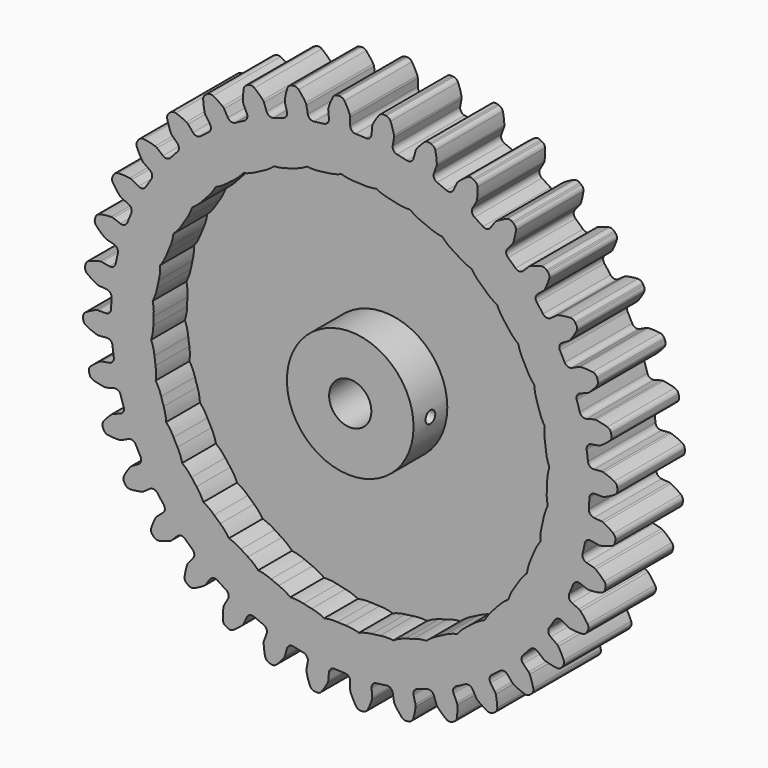
from build123d import *

# Parameters (mm, degrees)
F1_DEPTH = 12.7
F2_R     = 3.175
F3_DEPTH = 12.701
F4_T     = -6.35
F6_R     = 0.9144
F7_DEPTH = 9.525


# Not quite as in the source:
# - a shell that OpenCascade refuses in one call is made with other operations: the cavity is built on its own and cut out


with BuildPart() as f1:
    # F0 (on Front) → F1 (new body)
    with BuildSketch(Plane.XZ):
        with BuildLine():
            ThreePointArc((0, 37.9424051819), (-0.0153371145, 38.1007918887), (-0.0607785558, 38.2532932047))
            ThreePointArc((-0.0607785558, 38.2532932047), (-0.4269499275, 39.0474115053), (-0.8644079312, 39.8046009426))
            ThreePointArc((-0.8644079312, 39.8046009426), (-1.1764211516, 40.0905083584), (-1.58910835, 40.18423443))
            Line((-1.58910835, 40.18423443), (-1.7542226688, 40.1783047252))
            Line((-1.7542226688, 40.1783047252), (-1.9192254855, 40.1698212046))
            ThreePointArc((-1.9192254855, 40.1698212046), (-2.3221735191, 40.0404837297), (-2.6080809619, 39.7284705339))
            ThreePointArc((-2.6080809619, 39.7284705339), (-2.977880898, 38.9360354539), (-3.2734469068, 38.1130250753))
            ThreePointArc((-3.2734469068, 38.1130250753), (-3.3054240642, 37.9571435902), (-3.3068985053, 37.798022875))
            Line((-3.3068985053, 37.798022875), (-3.2072574352, 36.6591202325))
            ThreePointArc((-3.2072574352, 36.6591202325), (-3.3913357559, 36.0636768654), (-3.9392441989, 35.7666348321))
            Line((-3.9392441989, 35.7666348321), (-5.452068566, 35.5674677257))
            ThreePointArc((-5.452068566, 35.5674677257), (-6.058187617, 35.7125791572), (-6.3901057047, 36.2400903084))
            Line((-6.3901057047, 36.2400903084), (-6.5886295161, 37.365974791))
            ThreePointArc((-6.5886295161, 37.365974791), (-6.6312371884, 37.5192919859), (-6.7024698477, 37.6615856408))
            ThreePointArc((-6.7024698477, 37.6615856408), (-7.2009754492, 38.3800545087), (-7.7632720488, 39.0497767518))
            ThreePointArc((-7.7632720488, 39.0497767518), (-8.1201923891, 39.2771600644), (-8.5428853032, 39.2977998464))
            Line((-8.5428853032, 39.2977998464), (-8.704461482, 39.2632884266))
            Line((-8.704461482, 39.2632884266), (-8.8654843873, 39.2262813513))
            ThreePointArc((-8.8654843873, 39.2262813513), (-9.239851518, 39.0289376116), (-9.4672348615, 38.6720172909))
            ThreePointArc((-9.4672348615, 38.6720172909), (-9.6938117981, 37.8274059953), (-9.8419732426, 36.9655744948))
            ThreePointArc((-9.8419732426, 36.9655744948), (-9.8463960593, 36.8065084247), (-9.8202170781, 36.6495490767))
            Line((-9.8202170781, 36.6495490767), (-9.5243214113, 35.5452514147))
            ThreePointArc((-9.5243214113, 35.5452514147), (-9.6022055131, 34.9268893053), (-10.090209188, 34.5392167052))
            Line((-10.090209188, 34.5392167052), (-11.5454653485, 34.0803762003))
            ThreePointArc((-11.5454653485, 34.0803762003), (-12.1675744249, 34.1180315944), (-12.5860512811, 34.5798916949))
            Line((-12.5860512811, 34.5798916949), (-12.9770668584, 35.6541981643))
            ThreePointArc((-12.9770668584, 35.6541981643), (-13.0456504759, 35.7977873818), (-13.1405099849, 35.9255498549))
            ThreePointArc((-13.1405099849, 35.9255498549), (-13.7562029759, 36.546538977), (-14.4262530737, 37.1084448546))
            ThreePointArc((-14.4262530737, 37.1084448546), (-14.8172356899, 37.2703951371), (-15.2370910093, 37.2173215002))
            Line((-15.2370910093, 37.2173215002), (-15.3902196378, 37.1552769774))
            Line((-15.3902196378, 37.1552769774), (-15.5423700321, 37.0908707886))
            ThreePointArc((-15.5423700321, 37.0908707886), (-15.8767813042, 36.8315169737), (-16.0387316204, 36.4405343714))
            ThreePointArc((-16.0387316204, 36.4405343714), (-16.1152011319, 35.5694099471), (-16.1114562016, 34.6949436388))
            ThreePointArc((-16.1114562016, 34.6949436388), (-16.0881902927, 34.5375261256), (-16.0351533242, 34.3874972752))
            Line((-16.0351533242, 34.3874972752), (-15.5519937009, 33.3513581193))
            ThreePointArc((-15.5519937009, 33.3513581193), (-15.5213171147, 32.7288658876), (-15.9345882767, 32.2623419565))
            ThreePointArc((-15.9345882767, 32.2623419565), (-16.6150587927, 31.9172309793), (-17.2880590087, 31.5577696895))
            ThreePointArc((-17.2880590087, 31.5577696895), (-17.9072556409, 31.4868249062), (-18.3995760581, 31.8690005704))
            Line((-18.3995760581, 31.8690005704), (-18.9712025909, 32.8590867682))
            ThreePointArc((-18.9712025909, 32.8590867682), (-19.0636782751, 32.9885851227), (-19.1792823757, 33.0979344158))
            ThreePointArc((-19.1792823757, 33.0979344158), (-19.893455236, 33.6025753519), (-20.6508996989, 34.0395916382))
            ThreePointArc((-20.6508996989, 34.0395916382), (-21.0640647821, 34.1311881132), (-21.4683254155, 34.006013673))
            Line((-21.4683254155, 34.006013673), (-21.6083537576, 33.9183212386))
            Line((-21.6083537576, 33.9183212386), (-21.7470086284, 33.8284728859))
            ThreePointArc((-21.7470086284, 33.8284728859), (-22.0313031244, 33.5149893302), (-22.1228996351, 33.1018242549))
            ThreePointArc((-22.1228996351, 33.1018242549), (-22.0469382341, 32.2306553767), (-21.8914007168, 31.3701244769))
            ThreePointArc((-21.8914007168, 31.3701244769), (-21.841153005, 31.2191385721), (-21.7628695508, 31.08059877))
            Line((-21.7628695508, 31.08059877), (-21.1071265316, 30.1441006842))
            ThreePointArc((-21.1071265316, 30.1441006842), (-20.96882135, 29.5363924414), (-21.294802964, 29.005192273))
            ThreePointArc((-21.294802964, 29.005192273), (-21.9050077115, 28.5471618419), (-22.5053637442, 28.0762963158))
            ThreePointArc((-22.5053637442, 28.0762963158), (-23.1028339558, 27.8989069763), (-23.6540390273, 28.1897859902))
            Line((-23.6540390273, 28.1897859902), (-24.3889079326, 29.0655686481))
            ThreePointArc((-24.3889079326, 29.0655686481), (-24.5024658566, 29.1770413976), (-24.6353019766, 29.2646549879))
            ThreePointArc((-24.6353019766, 29.2646549879), (-25.4262549254, 29.6376144785), (-26.2480791867, 29.9364626548))
            ThreePointArc((-26.2480791867, 29.9364626548), (-26.6708729248, 29.9549222097), (-27.0472556174, 29.7614503283))
            Line((-27.0472556174, 29.7614503283), (-27.169928983, 29.6507744726))
            Line((-27.169928983, 29.6507744726), (-27.2908753719, 29.5382139526))
            ThreePointArc((-27.2908753719, 29.5382139526), (-27.5164149476, 29.1801256953), (-27.5348745391, 28.7573319588))
            ThreePointArc((-27.5348745391, 28.7573319588), (-27.3087902743, 27.9125886522), (-27.0061860988, 27.0921399567))
            ThreePointArc((-27.0061860988, 27.0921399567), (-26.9304833354, 26.9521732907), (-26.8293319986, 26.8293319986))
            Line((-26.8293319986, 26.8293319986), (-26.0209300033, 26.0209300033))
            ThreePointArc((-26.0209300033, 26.0209300033), (-25.7791985593, 25.446470657), (-26.0079858389, 24.8667344996))
            ThreePointArc((-26.0079858389, 24.8667344996), (-26.5293840555, 24.3097016375), (-27.0388543905, 23.7417388857))
            ThreePointArc((-27.0388543905, 23.7417388857), (-27.5964443516, 23.4632948755), (-28.1897859902, 23.6540390273))
            Line((-28.1897859902, 23.6540390273), (-29.0655686481, 24.3889079326))
            ThreePointArc((-29.0655686481, 24.3889079326), (-29.1967584119, 24.478968034), (-29.3427903931, 24.5421838268))
            ThreePointArc((-29.3427903931, 24.5421838268), (-30.1864907252, 24.7721296865), (-31.0477240705, 24.9237294022))
            ThreePointArc((-31.0477240705, 24.9237294022), (-31.4673000898, 24.8684911528), (-31.8043686439, 24.6126003753))
            Line((-31.8043686439, 24.6126003753), (-31.9059596648, 24.4823039282))
            Line((-31.9059596648, 24.4823039282), (-32.0055226772, 24.3504513354))
            ThreePointArc((-32.0055226772, 24.3504513354), (-32.1654544266, 23.958638707), (-32.1102162135, 23.5390626829))
            ThreePointArc((-32.1102162135, 23.5390626829), (-31.7408785409, 22.7464120459), (-31.300402182, 21.9909744733))
            ThreePointArc((-31.300402182, 21.9909744733), (-31.2015445572, 21.8662798623), (-31.08059877, 21.7628695508))
            Line((-31.08059877, 21.7628695508), (-30.1441006842, 21.1071265316))
            ThreePointArc((-30.1441006842, 21.1071265316), (-29.8062878653, 20.5833707383), (-29.9309292248, 19.9727135815))
            ThreePointArc((-29.9309292248, 19.9727135815), (-30.3476784895, 19.3336034502), (-30.7507831285, 18.6858007336))
            ThreePointArc((-30.7507831285, 18.6858007336), (-31.2515507502, 18.3147624328), (-31.8690005704, 18.3995760581))
            Line((-31.8690005704, 18.3995760581), (-32.8590867682, 18.9712025909))
            ThreePointArc((-32.8590867682, 18.9712025909), (-33.0039222371, 19.0371136136), (-33.1587129716, 19.074010829))
            ThreePointArc((-33.1587129716, 19.074010829), (-34.0295252794, 19.1539562693), (-34.9039995693, 19.1537012437))
            ThreePointArc((-34.9039995693, 19.1537012437), (-35.3076092648, 19.0264435763), (-35.595122023, 18.7159090145))
            Line((-35.595122023, 18.7159090145), (-35.6725439074, 18.5699509676))
            Line((-35.6725439074, 18.5699509676), (-35.7476983714, 18.4228125762))
            ThreePointArc((-35.7476983714, 18.4228125762), (-35.8371628493, 18.0091806053), (-35.7099052168, 17.6055708988))
            ThreePointArc((-35.7099052168, 17.6055708988), (-35.2085362747, 16.8890972198), (-34.6435713836, 16.2216243584))
            ThreePointArc((-34.6435713836, 16.2216243584), (-34.5245626363, 16.1159905852), (-34.3874972752, 16.0351533242))
            Line((-34.3874972752, 16.0351533242), (-33.3513581193, 15.5519937009))
            ThreePointArc((-33.3513581193, 15.5519937009), (-32.9277281972, 15.0948555154), (-32.9444364719, 14.471831868))
            ThreePointArc((-32.9444364719, 14.471831868), (-33.2438740692, 13.7700635053), (-33.5283648817, 13.0621039816))
            ThreePointArc((-33.5283648817, 13.0621039816), (-33.9570945933, 12.6097452014), (-34.5798916949, 12.5860512811))
            Line((-34.5798916949, 12.5860512811), (-35.6541981643, 12.9770668584))
            ThreePointArc((-35.6541981643, 12.9770668584), (-35.808278586, 13.0168261293), (-35.9671248356, 13.0262836642))
            ThreePointArc((-35.9671248356, 13.0262836642), (-36.8385899278, 12.9537995833), (-37.6997347036, 12.8016975651))
            ThreePointArc((-37.6997347036, 12.8016975651), (-38.0751145988, 12.6062871396), (-38.3043356314, 12.2505442291))
            Line((-38.3043356314, 12.2505442291), (-38.3552359546, 12.0933594436))
            Line((-38.3552359546, 12.0933594436), (-38.4036983399, 11.9354059794))
            ThreePointArc((-38.4036983399, 11.9354059794), (-38.4199772133, 11.512522664), (-38.2245668202, 11.1371427518))
            ThreePointArc((-38.2245668202, 11.1371427518), (-37.6064004502, 10.518615721), (-36.9341131993, 9.959388396))
            ThreePointArc((-36.9341131993, 9.959388396), (-36.79856935, 9.8760250892), (-36.6495490767, 9.8202170781))
            Line((-36.6495490767, 9.8202170781), (-35.5452514147, 9.5243214113))
            ThreePointArc((-35.5452514147, 9.5243214113), (-35.0486761701, 9.147690746), (-34.9569436875, 8.5312308663))
            ThreePointArc((-34.9569436875, 8.5312308663), (-35.1299713576, 7.7881271488), (-35.2872042343, 7.0415218098))
            ThreePointArc((-35.2872042343, 7.0415218098), (-35.6308693003, 6.5215872428), (-36.2400903084, 6.3901057047))
            Line((-36.2400903084, 6.3901057047), (-37.365974791, 6.5886295161))
            ThreePointArc((-37.365974791, 6.5886295161), (-37.5246185099, 6.6010289699), (-37.6826938117, 6.5827594618))
            ThreePointArc((-37.6826938117, 6.5827594618), (-38.5283326624, 6.3600482518), (-39.3499824758, 6.0607207841))
            ThreePointArc((-39.3499824758, 6.0607207841), (-39.6857268427, 5.8030950472), (-39.8496913846, 5.4129528563))
            Line((-39.8496913846, 5.4129528563), (-39.8725235659, 5.2493173126))
            Line((-39.8725235659, 5.2493173126), (-39.8928213675, 5.0853481115))
            ThreePointArc((-39.8928213675, 5.0853481115), (-39.8354200112, 4.6660625471), (-39.5777943034, 4.3303181579))
            ThreePointArc((-39.5777943034, 4.3303181579), (-38.8616131778, 3.8285314062), (-38.1024306749, 3.3945414568))
            ThreePointArc((-38.1024306749, 3.3945414568), (-37.954470155, 3.3359815684), (-37.798022875, 3.3068985053))
            Line((-37.798022875, 3.3068985053), (-36.6591202325, 3.2072574352))
            ThreePointArc((-36.6591202325, 3.2072574352), (-36.104687853, 2.9225780222), (-35.9073018583, 2.3314127318))
            ThreePointArc((-35.9073018583, 2.3314127318), (-35.9486622428, 1.5695524898), (-35.9738597423, 0.8069865611))
            ThreePointArc((-35.9738597423, 0.8069865611), (-36.2220180737, 0.235274156), (-36.7991521163, 0))
            Line((-36.7991521163, 0), (-37.9424051819, 0))
            ThreePointArc((-37.9424051819, 0), (-38.1007918887, -0.0153371145), (-38.2532932047, -0.0607785558))
            ThreePointArc((-38.2532932047, -0.0607785558), (-39.0474115053, -0.4269499275), (-39.8046009426, -0.8644079312))
            ThreePointArc((-39.8046009426, -0.8644079312), (-40.0905083584, -1.1764211516), (-40.18423443, -1.58910835))
            Line((-40.18423443, -1.58910835), (-40.1783047252, -1.7542226688))
            Line((-40.1783047252, -1.7542226688), (-40.1698212046, -1.9192254855))
            ThreePointArc((-40.1698212046, -1.9192254855), (-40.0404837297, -2.3221735191), (-39.7284705339, -2.6080809619))
            ThreePointArc((-39.7284705339, -2.6080809619), (-38.9360354539, -2.977880898), (-38.1130250753, -3.2734469068))
            ThreePointArc((-38.1130250753, -3.2734469068), (-37.9571435902, -3.3054240642), (-37.798022875, -3.3068985053))
            Line((-37.798022875, -3.3068985053), (-36.6591202325, -3.2072574352))
            ThreePointArc((-36.6591202325, -3.2072574352), (-36.0636768654, -3.3913357559), (-35.7666348321, -3.9392441989))
            ThreePointArc((-35.7666348321, -3.9392441989), (-35.6750712168, -4.6967122273), (-35.5674677257, -5.452068566))
            ThreePointArc((-35.5674677257, -5.452068566), (-35.7125791572, -6.058187617), (-36.2400903084, -6.3901057047))
            Line((-36.2400903084, -6.3901057047), (-37.365974791, -6.5886295161))
            ThreePointArc((-37.365974791, -6.5886295161), (-37.5192919859, -6.6312371884), (-37.6615856408, -6.7024698477))
            ThreePointArc((-37.6615856408, -6.7024698477), (-38.3800545087, -7.2009754492), (-39.0497767518, -7.7632720488))
            ThreePointArc((-39.0497767518, -7.7632720488), (-39.2771600644, -8.1201923891), (-39.2977998464, -8.5428853032))
            Line((-39.2977998464, -8.5428853032), (-39.2632884266, -8.704461482))
            Line((-39.2632884266, -8.704461482), (-39.2262813513, -8.8654843873))
            ThreePointArc((-39.2262813513, -8.8654843873), (-39.0289376116, -9.239851518), (-38.6720172909, -9.4672348615))
            ThreePointArc((-38.6720172909, -9.4672348615), (-37.8274059953, -9.6938117981), (-36.9655744948, -9.8419732426))
            ThreePointArc((-36.9655744948, -9.8419732426), (-36.8065084247, -9.8463960593), (-36.6495490767, -9.8202170781))
            Line((-36.6495490767, -9.8202170781), (-35.5452514147, -9.5243214113))
            ThreePointArc((-35.5452514147, -9.5243214113), (-34.9268893053, -9.6022055131), (-34.5392167052, -10.090209188))
            ThreePointArc((-34.5392167052, -10.090209188), (-34.3175112042, -10.82026972), (-34.0803762003, -11.5454653485))
            ThreePointArc((-34.0803762003, -11.5454653485), (-34.1180315944, -12.1675744249), (-34.5798916949, -12.5860512811))
            Line((-34.5798916949, -12.5860512811), (-35.6541981643, -12.9770668584))
            ThreePointArc((-35.6541981643, -12.9770668584), (-35.7977873818, -13.0456504759), (-35.9255498549, -13.1405099849))
            ThreePointArc((-35.9255498549, -13.1405099849), (-36.546538977, -13.7562029759), (-37.1084448546, -14.4262530737))
            ThreePointArc((-37.1084448546, -14.4262530737), (-37.2703951371, -14.8172356899), (-37.2173215002, -15.2370910093))
            Line((-37.2173215002, -15.2370910093), (-37.1552769774, -15.3902196378))
            Line((-37.1552769774, -15.3902196378), (-37.0908707886, -15.5423700321))
            ThreePointArc((-37.0908707886, -15.5423700321), (-36.8315169737, -15.8767813042), (-36.4405343714, -16.0387316204))
            ThreePointArc((-36.4405343714, -16.0387316204), (-35.5694099471, -16.1152011319), (-34.6949436388, -16.1114562016))
            ThreePointArc((-34.6949436388, -16.1114562016), (-34.5375261256, -16.0881902927), (-34.3874972752, -16.0351533242))
            Line((-34.3874972752, -16.0351533242), (-33.3513581193, -15.5519937009))
            ThreePointArc((-33.3513581193, -15.5519937009), (-32.7288658876, -15.5213171147), (-32.2623419565, -15.9345882767))
            ThreePointArc((-32.2623419565, -15.9345882767), (-31.9172309793, -16.6150587927), (-31.5577696895, -17.2880590087))
            ThreePointArc((-31.5577696895, -17.2880590087), (-31.4868249062, -17.9072556409), (-31.8690005704, -18.3995760581))
            Line((-31.8690005704, -18.3995760581), (-32.8590867682, -18.9712025909))
            ThreePointArc((-32.8590867682, -18.9712025909), (-32.9885851227, -19.0636782751), (-33.0979344158, -19.1792823757))
            ThreePointArc((-33.0979344158, -19.1792823757), (-33.6025753519, -19.893455236), (-34.0395916382, -20.6508996989))
            ThreePointArc((-34.0395916382, -20.6508996989), (-34.1311881132, -21.0640647821), (-34.006013673, -21.4683254155))
            Line((-34.006013673, -21.4683254155), (-33.9183212386, -21.6083537576))
            Line((-33.9183212386, -21.6083537576), (-33.8284728859, -21.7470086284))
            ThreePointArc((-33.8284728859, -21.7470086284), (-33.5149893302, -22.0313031244), (-33.1018242549, -22.1228996351))
            ThreePointArc((-33.1018242549, -22.1228996351), (-32.2306553767, -22.0469382341), (-31.3701244769, -21.8914007168))
            ThreePointArc((-31.3701244769, -21.8914007168), (-31.2191385721, -21.841153005), (-31.08059877, -21.7628695508))
            Line((-31.08059877, -21.7628695508), (-30.1441006842, -21.1071265316))
            ThreePointArc((-30.1441006842, -21.1071265316), (-29.5363924414, -20.96882135), (-29.005192273, -21.294802964))
            ThreePointArc((-29.005192273, -21.294802964), (-28.5471618419, -21.9050077115), (-28.0762963158, -22.5053637442))
            ThreePointArc((-28.0762963158, -22.5053637442), (-27.8989069763, -23.1028339558), (-28.1897859902, -23.6540390273))
            Line((-28.1897859902, -23.6540390273), (-29.0655686481, -24.3889079326))
            ThreePointArc((-29.0655686481, -24.3889079326), (-29.1770413976, -24.5024658566), (-29.2646549879, -24.6353019766))
            ThreePointArc((-29.2646549879, -24.6353019766), (-29.6376144785, -25.4262549254), (-29.9364626548, -26.2480791867))
            ThreePointArc((-29.9364626548, -26.2480791867), (-29.9549222097, -26.6708729248), (-29.7614503283, -27.0472556174))
            Line((-29.7614503283, -27.0472556174), (-29.6507744726, -27.169928983))
            Line((-29.6507744726, -27.169928983), (-29.5382139526, -27.2908753719))
            ThreePointArc((-29.5382139526, -27.2908753719), (-29.1801256953, -27.5164149476), (-28.7573319588, -27.5348745391))
            ThreePointArc((-28.7573319588, -27.5348745391), (-27.9125886522, -27.3087902743), (-27.0921399567, -27.0061860988))
            ThreePointArc((-27.0921399567, -27.0061860988), (-26.9521732907, -26.9304833354), (-26.8293319986, -26.8293319986))
            Line((-26.8293319986, -26.8293319986), (-26.0209300033, -26.0209300033))
            ThreePointArc((-26.0209300033, -26.0209300033), (-25.446470657, -25.7791985593), (-24.8667344996, -26.0079858389))
            ThreePointArc((-24.8667344996, -26.0079858389), (-24.3097016375, -26.5293840555), (-23.7417388857, -27.0388543905))
            ThreePointArc((-23.7417388857, -27.0388543905), (-23.4632948755, -27.5964443516), (-23.6540390273, -28.1897859902))
            Line((-23.6540390273, -28.1897859902), (-24.3889079326, -29.0655686481))
            ThreePointArc((-24.3889079326, -29.0655686481), (-24.478968034, -29.1967584119), (-24.5421838268, -29.3427903931))
            ThreePointArc((-24.5421838268, -29.3427903931), (-24.7721296865, -30.1864907252), (-24.9237294022, -31.0477240705))
            ThreePointArc((-24.9237294022, -31.0477240705), (-24.8684911528, -31.4673000898), (-24.6126003753, -31.8043686439))
            Line((-24.6126003753, -31.8043686439), (-24.4823039282, -31.9059596648))
            Line((-24.4823039282, -31.9059596648), (-24.3504513354, -32.0055226772))
            ThreePointArc((-24.3504513354, -32.0055226772), (-23.958638707, -32.1654544266), (-23.5390626829, -32.1102162135))
            ThreePointArc((-23.5390626829, -32.1102162135), (-22.7464120459, -31.7408785409), (-21.9909744733, -31.300402182))
            ThreePointArc((-21.9909744733, -31.300402182), (-21.8662798623, -31.2015445572), (-21.7628695508, -31.08059877))
            Line((-21.7628695508, -31.08059877), (-21.1071265316, -30.1441006842))
            ThreePointArc((-21.1071265316, -30.1441006842), (-20.5833707383, -29.8062878653), (-19.9727135815, -29.9309292248))
            ThreePointArc((-19.9727135815, -29.9309292248), (-19.3336034502, -30.3476784895), (-18.6858007336, -30.7507831285))
            ThreePointArc((-18.6858007336, -30.7507831285), (-18.3147624328, -31.2515507502), (-18.3995760581, -31.8690005704))
            Line((-18.3995760581, -31.8690005704), (-18.9712025909, -32.8590867682))
            ThreePointArc((-18.9712025909, -32.8590867682), (-19.0371136136, -33.0039222371), (-19.074010829, -33.1587129716))
            ThreePointArc((-19.074010829, -33.1587129716), (-19.1539562693, -34.0295252794), (-19.1537012437, -34.9039995693))
            ThreePointArc((-19.1537012437, -34.9039995693), (-19.0264435763, -35.3076092648), (-18.7159090145, -35.595122023))
            Line((-18.7159090145, -35.595122023), (-18.5699509676, -35.6725439074))
            Line((-18.5699509676, -35.6725439074), (-18.4228125762, -35.7476983714))
            ThreePointArc((-18.4228125762, -35.7476983714), (-18.0091806053, -35.8371628493), (-17.6055708988, -35.7099052168))
            ThreePointArc((-17.6055708988, -35.7099052168), (-16.8890972198, -35.2085362747), (-16.2216243584, -34.6435713836))
            ThreePointArc((-16.2216243584, -34.6435713836), (-16.1159905852, -34.5245626363), (-16.0351533242, -34.3874972752))
            Line((-16.0351533242, -34.3874972752), (-15.5519937009, -33.3513581193))
            ThreePointArc((-15.5519937009, -33.3513581193), (-15.0948555154, -32.9277281972), (-14.471831868, -32.9444364719))
            ThreePointArc((-14.471831868, -32.9444364719), (-13.7700635053, -33.2438740692), (-13.0621039816, -33.5283648817))
            ThreePointArc((-13.0621039816, -33.5283648817), (-12.6097452014, -33.9570945933), (-12.5860512811, -34.5798916949))
            Line((-12.5860512811, -34.5798916949), (-12.9770668584, -35.6541981643))
            ThreePointArc((-12.9770668584, -35.6541981643), (-13.0168261293, -35.808278586), (-13.0262836642, -35.9671248356))
            ThreePointArc((-13.0262836642, -35.9671248356), (-12.9537995833, -36.8385899278), (-12.8016975651, -37.6997347036))
            ThreePointArc((-12.8016975651, -37.6997347036), (-12.6062871396, -38.0751145988), (-12.2505442291, -38.3043356314))
            Line((-12.2505442291, -38.3043356314), (-12.0933594436, -38.3552359546))
            Line((-12.0933594436, -38.3552359546), (-11.9354059794, -38.4036983399))
            ThreePointArc((-11.9354059794, -38.4036983399), (-11.512522664, -38.4199772133), (-11.1371427518, -38.2245668202))
            ThreePointArc((-11.1371427518, -38.2245668202), (-10.518615721, -37.6064004502), (-9.959388396, -36.9341131993))
            ThreePointArc((-9.959388396, -36.9341131993), (-9.8760250892, -36.79856935), (-9.8202170781, -36.6495490767))
            Line((-9.8202170781, -36.6495490767), (-9.5243214113, -35.5452514147))
            ThreePointArc((-9.5243214113, -35.5452514147), (-9.147690746, -35.0486761701), (-8.5312308663, -34.9569436875))
            ThreePointArc((-8.5312308663, -34.9569436875), (-7.7881271488, -35.1299713576), (-7.0415218098, -35.2872042343))
            ThreePointArc((-7.0415218098, -35.2872042343), (-6.5215872428, -35.6308693003), (-6.3901057047, -36.2400903084))
            Line((-6.3901057047, -36.2400903084), (-6.5886295161, -37.365974791))
            ThreePointArc((-6.5886295161, -37.365974791), (-6.6010289699, -37.5246185099), (-6.5827594618, -37.6826938117))
            ThreePointArc((-6.5827594618, -37.6826938117), (-6.3600482518, -38.5283326624), (-6.0607207841, -39.3499824758))
            ThreePointArc((-6.0607207841, -39.3499824758), (-5.8030950472, -39.6857268427), (-5.4129528563, -39.8496913846))
            Line((-5.4129528563, -39.8496913846), (-5.2493173126, -39.8725235659))
            Line((-5.2493173126, -39.8725235659), (-5.0853481115, -39.8928213675))
            ThreePointArc((-5.0853481115, -39.8928213675), (-4.6660625471, -39.8354200112), (-4.3303181579, -39.5777943034))
            ThreePointArc((-4.3303181579, -39.5777943034), (-3.8285314062, -38.8616131778), (-3.3945414568, -38.1024306749))
            ThreePointArc((-3.3945414568, -38.1024306749), (-3.3359815684, -37.954470155), (-3.3068985053, -37.798022875))
            Line((-3.3068985053, -37.798022875), (-3.2072574352, -36.6591202325))
            ThreePointArc((-3.2072574352, -36.6591202325), (-2.9225780222, -36.104687853), (-2.3314127318, -35.9073018583))
            ThreePointArc((-2.3314127318, -35.9073018583), (-1.5695524898, -35.9486622428), (-0.8069865611, -35.9738597423))
            ThreePointArc((-0.8069865611, -35.9738597423), (-0.235274156, -36.2220180737), (0, -36.7991521163))
            Line((0, -36.7991521163), (0, -37.9424051819))
            ThreePointArc((0, -37.9424051819), (0.0153371145, -38.1007918887), (0.0607785558, -38.2532932047))
            ThreePointArc((0.0607785558, -38.2532932047), (0.4269499275, -39.0474115053), (0.8644079312, -39.8046009426))
            ThreePointArc((0.8644079312, -39.8046009426), (1.1764211516, -40.0905083584), (1.58910835, -40.18423443))
            Line((1.58910835, -40.18423443), (1.7542226688, -40.1783047252))
            Line((1.7542226688, -40.1783047252), (1.9192254855, -40.1698212046))
            ThreePointArc((1.9192254855, -40.1698212046), (2.3221735191, -40.0404837297), (2.6080809619, -39.7284705339))
            ThreePointArc((2.6080809619, -39.7284705339), (2.977880898, -38.9360354539), (3.2734469068, -38.1130250753))
            ThreePointArc((3.2734469068, -38.1130250753), (3.3054240642, -37.9571435902), (3.3068985053, -37.798022875))
            Line((3.3068985053, -37.798022875), (3.2072574352, -36.6591202325))
            ThreePointArc((3.2072574352, -36.6591202325), (3.3913357559, -36.0636768654), (3.9392441989, -35.7666348321))
            ThreePointArc((3.9392441989, -35.7666348321), (4.6967122273, -35.6750712168), (5.452068566, -35.5674677257))
            ThreePointArc((5.452068566, -35.5674677257), (6.058187617, -35.7125791572), (6.3901057047, -36.2400903084))
            Line((6.3901057047, -36.2400903084), (6.5886295161, -37.365974791))
            ThreePointArc((6.5886295161, -37.365974791), (6.6312371884, -37.5192919859), (6.7024698477, -37.6615856408))
            ThreePointArc((6.7024698477, -37.6615856408), (7.2009754492, -38.3800545087), (7.7632720488, -39.0497767518))
            ThreePointArc((7.7632720488, -39.0497767518), (8.1201923891, -39.2771600644), (8.5428853032, -39.2977998464))
            Line((8.5428853032, -39.2977998464), (8.704461482, -39.2632884266))
            Line((8.704461482, -39.2632884266), (8.8654843873, -39.2262813513))
            ThreePointArc((8.8654843873, -39.2262813513), (9.239851518, -39.0289376116), (9.4672348615, -38.6720172909))
            ThreePointArc((9.4672348615, -38.6720172909), (9.6938117981, -37.8274059953), (9.8419732426, -36.9655744948))
            ThreePointArc((9.8419732426, -36.9655744948), (9.8463960593, -36.8065084247), (9.8202170781, -36.6495490767))
            Line((9.8202170781, -36.6495490767), (9.5243214113, -35.5452514147))
            ThreePointArc((9.5243214113, -35.5452514147), (9.6022055131, -34.9268893053), (10.090209188, -34.5392167052))
            ThreePointArc((10.090209188, -34.5392167052), (10.82026972, -34.3175112042), (11.5454653485, -34.0803762003))
            ThreePointArc((11.5454653485, -34.0803762003), (12.1675744249, -34.1180315944), (12.5860512811, -34.5798916949))
            Line((12.5860512811, -34.5798916949), (12.9770668584, -35.6541981643))
            ThreePointArc((12.9770668584, -35.6541981643), (13.0456504759, -35.7977873818), (13.1405099849, -35.9255498549))
            ThreePointArc((13.1405099849, -35.9255498549), (13.7562029759, -36.546538977), (14.4262530737, -37.1084448546))
            ThreePointArc((14.4262530737, -37.1084448546), (14.8172356899, -37.2703951371), (15.2370910093, -37.2173215002))
            Line((15.2370910093, -37.2173215002), (15.3902196378, -37.1552769774))
            Line((15.3902196378, -37.1552769774), (15.5423700321, -37.0908707886))
            ThreePointArc((15.5423700321, -37.0908707886), (15.8767813042, -36.8315169737), (16.0387316204, -36.4405343714))
            ThreePointArc((16.0387316204, -36.4405343714), (16.1152011319, -35.5694099471), (16.1114562016, -34.6949436388))
            ThreePointArc((16.1114562016, -34.6949436388), (16.0881902927, -34.5375261256), (16.0351533242, -34.3874972752))
            Line((16.0351533242, -34.3874972752), (15.5519937009, -33.3513581193))
            ThreePointArc((15.5519937009, -33.3513581193), (15.5213171147, -32.7288658876), (15.9345882767, -32.2623419565))
            ThreePointArc((15.9345882767, -32.2623419565), (16.6150587927, -31.9172309793), (17.2880590087, -31.5577696895))
            ThreePointArc((17.2880590087, -31.5577696895), (17.9072556409, -31.4868249062), (18.3995760581, -31.8690005704))
            Line((18.3995760581, -31.8690005704), (18.9712025909, -32.8590867682))
            ThreePointArc((18.9712025909, -32.8590867682), (19.0636782751, -32.9885851227), (19.1792823757, -33.0979344158))
            ThreePointArc((19.1792823757, -33.0979344158), (19.893455236, -33.6025753519), (20.6508996989, -34.0395916382))
            ThreePointArc((20.6508996989, -34.0395916382), (21.0640647821, -34.1311881132), (21.4683254155, -34.006013673))
            Line((21.4683254155, -34.006013673), (21.6083537576, -33.9183212386))
            Line((21.6083537576, -33.9183212386), (21.7470086284, -33.8284728859))
            ThreePointArc((21.7470086284, -33.8284728859), (22.0313031244, -33.5149893302), (22.1228996351, -33.1018242549))
            ThreePointArc((22.1228996351, -33.1018242549), (22.0469382341, -32.2306553767), (21.8914007168, -31.3701244769))
            ThreePointArc((21.8914007168, -31.3701244769), (21.841153005, -31.2191385721), (21.7628695508, -31.08059877))
            Line((21.7628695508, -31.08059877), (21.1071265316, -30.1441006842))
            ThreePointArc((21.1071265316, -30.1441006842), (20.96882135, -29.5363924414), (21.294802964, -29.005192273))
            ThreePointArc((21.294802964, -29.005192273), (21.9050077115, -28.5471618419), (22.5053637442, -28.0762963158))
            ThreePointArc((22.5053637442, -28.0762963158), (23.1028339558, -27.8989069763), (23.6540390273, -28.1897859902))
            Line((23.6540390273, -28.1897859902), (24.3889079326, -29.0655686481))
            ThreePointArc((24.3889079326, -29.0655686481), (24.5024658566, -29.1770413976), (24.6353019766, -29.2646549879))
            ThreePointArc((24.6353019766, -29.2646549879), (25.4262549254, -29.6376144785), (26.2480791867, -29.9364626548))
            ThreePointArc((26.2480791867, -29.9364626548), (26.6708729248, -29.9549222097), (27.0472556174, -29.7614503283))
            Line((27.0472556174, -29.7614503283), (27.169928983, -29.6507744726))
            Line((27.169928983, -29.6507744726), (27.2908753719, -29.5382139526))
            ThreePointArc((27.2908753719, -29.5382139526), (27.5164149476, -29.1801256953), (27.5348745391, -28.7573319588))
            ThreePointArc((27.5348745391, -28.7573319588), (27.3087902743, -27.9125886522), (27.0061860988, -27.0921399567))
            ThreePointArc((27.0061860988, -27.0921399567), (26.9304833354, -26.9521732907), (26.8293319986, -26.8293319986))
            Line((26.8293319986, -26.8293319986), (26.0209300033, -26.0209300033))
            ThreePointArc((26.0209300033, -26.0209300033), (25.7791985593, -25.446470657), (26.0079858389, -24.8667344996))
            ThreePointArc((26.0079858389, -24.8667344996), (26.5293840555, -24.3097016375), (27.0388543905, -23.7417388857))
            ThreePointArc((27.0388543905, -23.7417388857), (27.5964443516, -23.4632948755), (28.1897859902, -23.6540390273))
            Line((28.1897859902, -23.6540390273), (29.0655686481, -24.3889079326))
            ThreePointArc((29.0655686481, -24.3889079326), (29.1967584119, -24.478968034), (29.3427903931, -24.5421838268))
            ThreePointArc((29.3427903931, -24.5421838268), (30.1864907252, -24.7721296865), (31.0477240705, -24.9237294022))
            ThreePointArc((31.0477240705, -24.9237294022), (31.4673000898, -24.8684911528), (31.8043686439, -24.6126003753))
            Line((31.8043686439, -24.6126003753), (31.9059596648, -24.4823039282))
            Line((31.9059596648, -24.4823039282), (32.0055226772, -24.3504513354))
            ThreePointArc((32.0055226772, -24.3504513354), (32.1654544266, -23.958638707), (32.1102162135, -23.5390626829))
            ThreePointArc((32.1102162135, -23.5390626829), (31.7408785409, -22.7464120459), (31.300402182, -21.9909744733))
            ThreePointArc((31.300402182, -21.9909744733), (31.2015445572, -21.8662798623), (31.08059877, -21.7628695508))
            Line((31.08059877, -21.7628695508), (30.1441006842, -21.1071265316))
            ThreePointArc((30.1441006842, -21.1071265316), (29.8062878653, -20.5833707383), (29.9309292248, -19.9727135815))
            ThreePointArc((29.9309292248, -19.9727135815), (30.3476784895, -19.3336034502), (30.7507831285, -18.6858007336))
            ThreePointArc((30.7507831285, -18.6858007336), (31.2515507502, -18.3147624328), (31.8690005704, -18.3995760581))
            Line((31.8690005704, -18.3995760581), (32.8590867682, -18.9712025909))
            ThreePointArc((32.8590867682, -18.9712025909), (33.0039222371, -19.0371136136), (33.1587129716, -19.074010829))
            ThreePointArc((33.1587129716, -19.074010829), (34.0295252794, -19.1539562693), (34.9039995693, -19.1537012437))
            ThreePointArc((34.9039995693, -19.1537012437), (35.3076092648, -19.0264435763), (35.595122023, -18.7159090145))
            Line((35.595122023, -18.7159090145), (35.6725439074, -18.5699509676))
            Line((35.6725439074, -18.5699509676), (35.7476983714, -18.4228125762))
            ThreePointArc((35.7476983714, -18.4228125762), (35.8371628493, -18.0091806053), (35.7099052168, -17.6055708988))
            ThreePointArc((35.7099052168, -17.6055708988), (35.2085362747, -16.8890972198), (34.6435713836, -16.2216243584))
            ThreePointArc((34.6435713836, -16.2216243584), (34.5245626363, -16.1159905852), (34.3874972752, -16.0351533242))
            Line((34.3874972752, -16.0351533242), (33.3513581193, -15.5519937009))
            ThreePointArc((33.3513581193, -15.5519937009), (32.9277281972, -15.0948555154), (32.9444364719, -14.471831868))
            ThreePointArc((32.9444364719, -14.471831868), (33.2438740692, -13.7700635053), (33.5283648817, -13.0621039816))
            ThreePointArc((33.5283648817, -13.0621039816), (33.9570945933, -12.6097452014), (34.5798916949, -12.5860512811))
            Line((34.5798916949, -12.5860512811), (35.6541981643, -12.9770668584))
            ThreePointArc((35.6541981643, -12.9770668584), (35.808278586, -13.0168261293), (35.9671248356, -13.0262836642))
            ThreePointArc((35.9671248356, -13.0262836642), (36.8385899278, -12.9537995833), (37.6997347036, -12.8016975651))
            ThreePointArc((37.6997347036, -12.8016975651), (38.0751145988, -12.6062871396), (38.3043356314, -12.2505442291))
            Line((38.3043356314, -12.2505442291), (38.3552359546, -12.0933594436))
            Line((38.3552359546, -12.0933594436), (38.4036983399, -11.9354059794))
            ThreePointArc((38.4036983399, -11.9354059794), (38.4199772133, -11.512522664), (38.2245668202, -11.1371427518))
            ThreePointArc((38.2245668202, -11.1371427518), (37.6064004502, -10.518615721), (36.9341131993, -9.959388396))
            ThreePointArc((36.9341131993, -9.959388396), (36.79856935, -9.8760250892), (36.6495490767, -9.8202170781))
            Line((36.6495490767, -9.8202170781), (35.5452514147, -9.5243214113))
            ThreePointArc((35.5452514147, -9.5243214113), (35.0486761701, -9.147690746), (34.9569436875, -8.5312308663))
            ThreePointArc((34.9569436875, -8.5312308663), (35.1299713576, -7.7881271488), (35.2872042343, -7.0415218098))
            ThreePointArc((35.2872042343, -7.0415218098), (35.6308693003, -6.5215872428), (36.2400903084, -6.3901057047))
            Line((36.2400903084, -6.3901057047), (37.365974791, -6.5886295161))
            ThreePointArc((37.365974791, -6.5886295161), (37.5246185099, -6.6010289699), (37.6826938117, -6.5827594618))
            ThreePointArc((37.6826938117, -6.5827594618), (38.5283326624, -6.3600482518), (39.3499824758, -6.0607207841))
            ThreePointArc((39.3499824758, -6.0607207841), (39.6857268427, -5.8030950472), (39.8496913846, -5.4129528563))
            Line((39.8496913846, -5.4129528563), (39.8725235659, -5.2493173126))
            Line((39.8725235659, -5.2493173126), (39.8928213675, -5.0853481115))
            ThreePointArc((39.8928213675, -5.0853481115), (39.8354200112, -4.6660625471), (39.5777943034, -4.3303181579))
            ThreePointArc((39.5777943034, -4.3303181579), (38.8616131778, -3.8285314062), (38.1024306749, -3.3945414568))
            ThreePointArc((38.1024306749, -3.3945414568), (37.954470155, -3.3359815684), (37.798022875, -3.3068985053))
            Line((37.798022875, -3.3068985053), (36.6591202325, -3.2072574352))
            ThreePointArc((36.6591202325, -3.2072574352), (36.104687853, -2.9225780222), (35.9073018583, -2.3314127318))
            ThreePointArc((35.9073018583, -2.3314127318), (35.9486622428, -1.5695524898), (35.9738597423, -0.8069865611))
            ThreePointArc((35.9738597423, -0.8069865611), (36.2220180737, -0.235274156), (36.7991521163, 0))
            Line((36.7991521163, 0), (37.9424051819, 0))
            ThreePointArc((37.9424051819, 0), (38.1007918887, 0.0153371145), (38.2532932047, 0.0607785558))
            ThreePointArc((38.2532932047, 0.0607785558), (39.0474115053, 0.4269499275), (39.8046009426, 0.8644079312))
            ThreePointArc((39.8046009426, 0.8644079312), (40.0905083584, 1.1764211516), (40.18423443, 1.58910835))
            Line((40.18423443, 1.58910835), (40.1783047252, 1.7542226688))
            Line((40.1783047252, 1.7542226688), (40.1698212046, 1.9192254855))
            ThreePointArc((40.1698212046, 1.9192254855), (40.0404837297, 2.3221735191), (39.7284705339, 2.6080809619))
            ThreePointArc((39.7284705339, 2.6080809619), (38.9360354539, 2.977880898), (38.1130250753, 3.2734469068))
            ThreePointArc((38.1130250753, 3.2734469068), (37.9571435902, 3.3054240642), (37.798022875, 3.3068985053))
            Line((37.798022875, 3.3068985053), (36.6591202325, 3.2072574352))
            ThreePointArc((36.6591202325, 3.2072574352), (36.0636768654, 3.3913357559), (35.7666348321, 3.9392441989))
            ThreePointArc((35.7666348321, 3.9392441989), (35.6750712168, 4.6967122273), (35.5674677257, 5.452068566))
            ThreePointArc((35.5674677257, 5.452068566), (35.7125791572, 6.058187617), (36.2400903084, 6.3901057047))
            Line((36.2400903084, 6.3901057047), (37.365974791, 6.5886295161))
            ThreePointArc((37.365974791, 6.5886295161), (37.5192919859, 6.6312371884), (37.6615856408, 6.7024698477))
            ThreePointArc((37.6615856408, 6.7024698477), (38.3800545087, 7.2009754492), (39.0497767518, 7.7632720488))
            ThreePointArc((39.0497767518, 7.7632720488), (39.2771600644, 8.1201923891), (39.2977998464, 8.5428853032))
            Line((39.2977998464, 8.5428853032), (39.2632884266, 8.704461482))
            Line((39.2632884266, 8.704461482), (39.2262813513, 8.8654843873))
            ThreePointArc((39.2262813513, 8.8654843873), (39.0289376116, 9.239851518), (38.6720172909, 9.4672348615))
            ThreePointArc((38.6720172909, 9.4672348615), (37.8274059953, 9.6938117981), (36.9655744948, 9.8419732426))
            ThreePointArc((36.9655744948, 9.8419732426), (36.8065084247, 9.8463960593), (36.6495490767, 9.8202170781))
            Line((36.6495490767, 9.8202170781), (35.5452514147, 9.5243214113))
            ThreePointArc((35.5452514147, 9.5243214113), (34.9268893053, 9.6022055131), (34.5392167052, 10.090209188))
            ThreePointArc((34.5392167052, 10.090209188), (34.3175112042, 10.82026972), (34.0803762003, 11.5454653485))
            ThreePointArc((34.0803762003, 11.5454653485), (34.1180315944, 12.1675744249), (34.5798916949, 12.5860512811))
            Line((34.5798916949, 12.5860512811), (35.6541981643, 12.9770668584))
            ThreePointArc((35.6541981643, 12.9770668584), (35.7977873818, 13.0456504759), (35.9255498549, 13.1405099849))
            ThreePointArc((35.9255498549, 13.1405099849), (36.546538977, 13.7562029759), (37.1084448546, 14.4262530737))
            ThreePointArc((37.1084448546, 14.4262530737), (37.2703951371, 14.8172356899), (37.2173215002, 15.2370910093))
            Line((37.2173215002, 15.2370910093), (37.1552769774, 15.3902196378))
            Line((37.1552769774, 15.3902196378), (37.0908707886, 15.5423700321))
            ThreePointArc((37.0908707886, 15.5423700321), (36.8315169737, 15.8767813042), (36.4405343714, 16.0387316204))
            ThreePointArc((36.4405343714, 16.0387316204), (35.5694099471, 16.1152011319), (34.6949436388, 16.1114562016))
            ThreePointArc((34.6949436388, 16.1114562016), (34.5375261256, 16.0881902927), (34.3874972752, 16.0351533242))
            Line((34.3874972752, 16.0351533242), (33.3513581193, 15.5519937009))
            ThreePointArc((33.3513581193, 15.5519937009), (32.7288658876, 15.5213171147), (32.2623419565, 15.9345882767))
            ThreePointArc((32.2623419565, 15.9345882767), (31.9172309793, 16.6150587927), (31.5577696895, 17.2880590087))
            ThreePointArc((31.5577696895, 17.2880590087), (31.4868249062, 17.9072556409), (31.8690005704, 18.3995760581))
            Line((31.8690005704, 18.3995760581), (32.8590867682, 18.9712025909))
            ThreePointArc((32.8590867682, 18.9712025909), (32.9885851227, 19.0636782751), (33.0979344158, 19.1792823757))
            ThreePointArc((33.0979344158, 19.1792823757), (33.6025753519, 19.893455236), (34.0395916382, 20.6508996989))
            ThreePointArc((34.0395916382, 20.6508996989), (34.1311881132, 21.0640647821), (34.006013673, 21.4683254155))
            Line((34.006013673, 21.4683254155), (33.9183212386, 21.6083537576))
            Line((33.9183212386, 21.6083537576), (33.8284728859, 21.7470086284))
            ThreePointArc((33.8284728859, 21.7470086284), (33.5149893302, 22.0313031244), (33.1018242549, 22.1228996351))
            ThreePointArc((33.1018242549, 22.1228996351), (32.2306553767, 22.0469382341), (31.3701244769, 21.8914007168))
            ThreePointArc((31.3701244769, 21.8914007168), (31.2191385721, 21.841153005), (31.08059877, 21.7628695508))
            Line((31.08059877, 21.7628695508), (30.1441006842, 21.1071265316))
            ThreePointArc((30.1441006842, 21.1071265316), (29.5363924414, 20.96882135), (29.005192273, 21.294802964))
            ThreePointArc((29.005192273, 21.294802964), (28.5471618419, 21.9050077115), (28.0762963158, 22.5053637442))
            ThreePointArc((28.0762963158, 22.5053637442), (27.8989069763, 23.1028339558), (28.1897859902, 23.6540390273))
            Line((28.1897859902, 23.6540390273), (29.0655686481, 24.3889079326))
            ThreePointArc((29.0655686481, 24.3889079326), (29.1770413976, 24.5024658566), (29.2646549879, 24.6353019766))
            ThreePointArc((29.2646549879, 24.6353019766), (29.6376144785, 25.4262549254), (29.9364626548, 26.2480791867))
            ThreePointArc((29.9364626548, 26.2480791867), (29.9549222097, 26.6708729248), (29.7614503283, 27.0472556174))
            Line((29.7614503283, 27.0472556174), (29.6507744726, 27.169928983))
            Line((29.6507744726, 27.169928983), (29.5382139526, 27.2908753719))
            ThreePointArc((29.5382139526, 27.2908753719), (29.1801256953, 27.5164149476), (28.7573319588, 27.5348745391))
            ThreePointArc((28.7573319588, 27.5348745391), (27.9125886522, 27.3087902743), (27.0921399567, 27.0061860988))
            ThreePointArc((27.0921399567, 27.0061860988), (26.9521732907, 26.9304833354), (26.8293319986, 26.8293319986))
            Line((26.8293319986, 26.8293319986), (26.0209300033, 26.0209300033))
            ThreePointArc((26.0209300033, 26.0209300033), (25.446470657, 25.7791985593), (24.8667344996, 26.0079858389))
            ThreePointArc((24.8667344996, 26.0079858389), (24.3097016375, 26.5293840555), (23.7417388857, 27.0388543905))
            ThreePointArc((23.7417388857, 27.0388543905), (23.4632948755, 27.5964443516), (23.6540390273, 28.1897859902))
            Line((23.6540390273, 28.1897859902), (24.3889079326, 29.0655686481))
            ThreePointArc((24.3889079326, 29.0655686481), (24.478968034, 29.1967584119), (24.5421838268, 29.3427903931))
            ThreePointArc((24.5421838268, 29.3427903931), (24.7721296865, 30.1864907252), (24.9237294022, 31.0477240705))
            ThreePointArc((24.9237294022, 31.0477240705), (24.8684911528, 31.4673000898), (24.6126003753, 31.8043686439))
            Line((24.6126003753, 31.8043686439), (24.4823039282, 31.9059596648))
            Line((24.4823039282, 31.9059596648), (24.3504513354, 32.0055226772))
            ThreePointArc((24.3504513354, 32.0055226772), (23.958638707, 32.1654544266), (23.5390626829, 32.1102162135))
            ThreePointArc((23.5390626829, 32.1102162135), (22.7464120459, 31.7408785409), (21.9909744733, 31.300402182))
            ThreePointArc((21.9909744733, 31.300402182), (21.8662798623, 31.2015445572), (21.7628695508, 31.08059877))
            Line((21.7628695508, 31.08059877), (21.1071265316, 30.1441006842))
            ThreePointArc((21.1071265316, 30.1441006842), (20.5833707383, 29.8062878653), (19.9727135815, 29.9309292248))
            ThreePointArc((19.9727135815, 29.9309292248), (19.3336034502, 30.3476784895), (18.6858007336, 30.7507831285))
            ThreePointArc((18.6858007336, 30.7507831285), (18.3147624328, 31.2515507502), (18.3995760581, 31.8690005704))
            Line((18.3995760581, 31.8690005704), (18.9712025909, 32.8590867682))
            ThreePointArc((18.9712025909, 32.8590867682), (19.0371136136, 33.0039222371), (19.074010829, 33.1587129716))
            ThreePointArc((19.074010829, 33.1587129716), (19.1539562693, 34.0295252794), (19.1537012437, 34.9039995693))
            ThreePointArc((19.1537012437, 34.9039995693), (19.0264435763, 35.3076092648), (18.7159090145, 35.595122023))
            Line((18.7159090145, 35.595122023), (18.5699509676, 35.6725439074))
            Line((18.5699509676, 35.6725439074), (18.4228125762, 35.7476983714))
            ThreePointArc((18.4228125762, 35.7476983714), (18.0091806053, 35.8371628493), (17.6055708988, 35.7099052168))
            ThreePointArc((17.6055708988, 35.7099052168), (16.8890972198, 35.2085362747), (16.2216243584, 34.6435713836))
            ThreePointArc((16.2216243584, 34.6435713836), (16.1159905852, 34.5245626363), (16.0351533242, 34.3874972752))
            Line((16.0351533242, 34.3874972752), (15.5519937009, 33.3513581193))
            ThreePointArc((15.5519937009, 33.3513581193), (15.0948555154, 32.9277281972), (14.471831868, 32.9444364719))
            ThreePointArc((14.471831868, 32.9444364719), (13.7700635053, 33.2438740692), (13.0621039816, 33.5283648817))
            ThreePointArc((13.0621039816, 33.5283648817), (12.6097452014, 33.9570945933), (12.5860512811, 34.5798916949))
            Line((12.5860512811, 34.5798916949), (12.9770668584, 35.6541981643))
            ThreePointArc((12.9770668584, 35.6541981643), (13.0168261293, 35.808278586), (13.0262836642, 35.9671248356))
            ThreePointArc((13.0262836642, 35.9671248356), (12.9537995833, 36.8385899278), (12.8016975651, 37.6997347036))
            ThreePointArc((12.8016975651, 37.6997347036), (12.6062871396, 38.0751145988), (12.2505442291, 38.3043356314))
            Line((12.2505442291, 38.3043356314), (12.0933594436, 38.3552359546))
            Line((12.0933594436, 38.3552359546), (11.9354059794, 38.4036983399))
            ThreePointArc((11.9354059794, 38.4036983399), (11.512522664, 38.4199772133), (11.1371427518, 38.2245668202))
            ThreePointArc((11.1371427518, 38.2245668202), (10.518615721, 37.6064004502), (9.959388396, 36.9341131993))
            ThreePointArc((9.959388396, 36.9341131993), (9.8760250892, 36.79856935), (9.8202170781, 36.6495490767))
            Line((9.8202170781, 36.6495490767), (9.5243214113, 35.5452514147))
            ThreePointArc((9.5243214113, 35.5452514147), (9.147690746, 35.0486761701), (8.5312308663, 34.9569436875))
            Line((8.5312308663, 34.9569436875), (7.0415218098, 35.2872042343))
            ThreePointArc((7.0415218098, 35.2872042343), (6.5215872428, 35.6308693003), (6.3901057047, 36.2400903084))
            Line((6.3901057047, 36.2400903084), (6.5886295161, 37.365974791))
            ThreePointArc((6.5886295161, 37.365974791), (6.6010289699, 37.5246185099), (6.5827594618, 37.6826938117))
            ThreePointArc((6.5827594618, 37.6826938117), (6.3600482518, 38.5283326624), (6.0607207841, 39.3499824758))
            ThreePointArc((6.0607207841, 39.3499824758), (5.8030950472, 39.6857268427), (5.4129528563, 39.8496913846))
            Line((5.4129528563, 39.8496913846), (5.2493173126, 39.8725235659))
            Line((5.2493173126, 39.8725235659), (5.0853481115, 39.8928213675))
            ThreePointArc((5.0853481115, 39.8928213675), (4.6660625471, 39.8354200112), (4.3303181579, 39.5777943034))
            ThreePointArc((4.3303181579, 39.5777943034), (3.8285314062, 38.8616131778), (3.3945414568, 38.1024306749))
            ThreePointArc((3.3945414568, 38.1024306749), (3.3359815684, 37.954470155), (3.3068985053, 37.798022875))
            Line((3.3068985053, 37.798022875), (3.2072574352, 36.6591202325))
            ThreePointArc((3.2072574352, 36.6591202325), (2.9225780222, 36.104687853), (2.3314127318, 35.9073018583))
            ThreePointArc((2.3314127318, 35.9073018583), (1.5695524898, 35.9486622428), (0.8069865611, 35.9738597423))
            ThreePointArc((0.8069865611, 35.9738597423), (0.235274156, 36.2220180737), (0, 36.7991521163))
            Line((0, 36.7991521163), (0, 37.9424051819))
        make_face()
    extrude(amount=F1_DEPTH)

    # F2 (on face) → F3 (cut, through all)
    with BuildSketch(Plane.XZ.offset(12.7)):
        Circle(F2_R)
    extrude(amount=-F3_DEPTH, mode=Mode.SUBTRACT)

    # F4: a shell. OpenCascade refuses it in one call, so the cavity is built on its own and cut out:
    # the body offset inwards by the wall thickness, plus a prism from it out through each open face.
    f4_core = offset(f1.part, amount=F4_T, mode=Mode.PRIVATE)
    f4_exits = [f4_core.faces().sort_by_distance(p)[0] for p in [
        (-28.812821, -6.35, -2.049492),
    ]]
    add(f4_core, mode=Mode.SUBTRACT)
    extrude(f4_exits, amount=-F4_T, mode=Mode.SUBTRACT)

    # F6 (on offset) → F7 (cut)
    with BuildSketch(Plane.YZ.offset(9.525)):
        with Locations((-9.525, 0)):
            Circle(F6_R)
    extrude(amount=-F7_DEPTH, mode=Mode.SUBTRACT)


solid = f1.part
